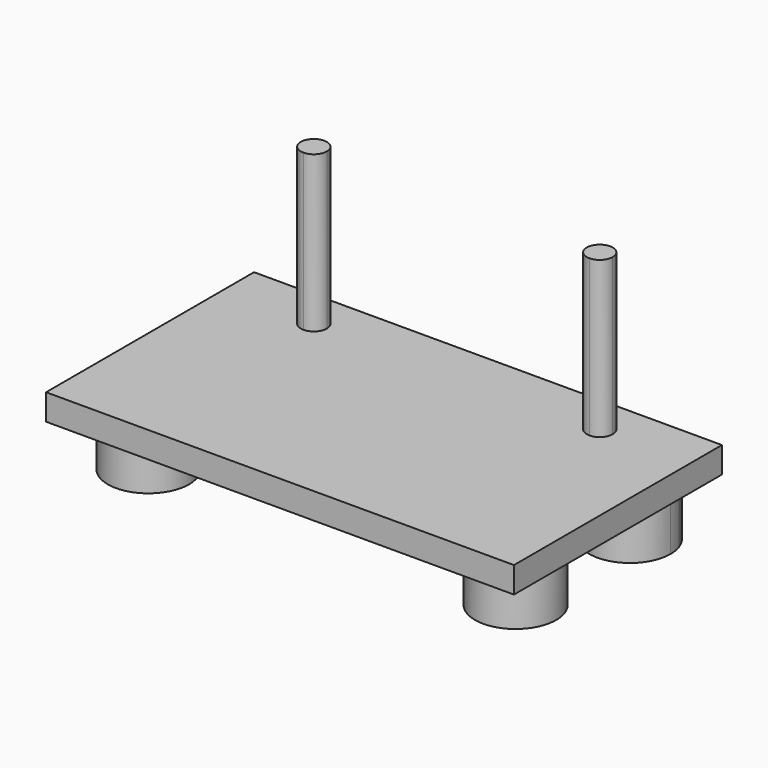
from build123d import *

# Parameters (mm, degrees)
F0_R     = 39.6875
F1_DEPTH = 25.4
F2_DEPTH = 76.2
F3_DEPTH = 152.4


with BuildPart() as f1:
    # F0 (on Top) → F1 (new body)
    with BuildSketch(Plane.XY):
        with BuildLine():
            Line((64.5657867546, -73.7079969396), (0, -73.7079969396))
            Line((0, -73.7079969396), (0, -213.4079969396))
            Line((0, -213.4079969396), (0, -276.9079969396))
            Line((0, -276.9079969396), (228.6, -276.9079969396))
            Line((228.6, -276.9079969396), (228.6, -61.0079969396))
            Line((228.6, -61.0079969396), (216.9881337214, -61.0079969396))
            ThreePointArc((216.9881337214, -61.0079969396), (218.5498084551, -67.2728393878), (219.075, -73.7079969396))
            ThreePointArc((219.075, -73.7079969396), (213.9674206511, -93.1843093218), (199.9593215616, -107.6476170595))
            ThreePointArc((199.9593215616, -107.6476170595), (121.1719117521, -134.9211212537), (64.5657867546, -73.7079969396))
        make_face()
        with BuildLine():
            ThreePointArc((219.075, -213.4079969396), (179.3875, -253.0954969396), (139.7, -213.4079969396))
            ThreePointArc((139.7, -213.4079969396), (179.3875, -173.7204969396), (219.075, -213.4079969396))
        make_face(mode=Mode.SUBTRACT)
        with BuildLine():
            Line((0, -213.4079969396), (0, -73.7079969396))
            Line((0, -73.7079969396), (-64.5657867546, -73.7079969396))
            ThreePointArc((-64.5657867546, -73.7079969396), (-121.1719117521, -134.9211212537), (-199.9593215616, -107.6476170595))
            ThreePointArc((-199.9593215616, -107.6476170595), (-216.6678189317, -87.3195904026), (-216.9881337214, -61.0079969396))
            Line((-216.9881337214, -61.0079969396), (-228.6, -61.0079969396))
            Line((-228.6, -61.0079969396), (-228.6, -276.9079969396))
            Line((-228.6, -276.9079969396), (0, -276.9079969396))
            Line((0, -276.9079969396), (0, -213.4079969396))
        make_face()
        with Locations((-179.3875, -213.4079969396)):
            Circle(F0_R, mode=Mode.SUBTRACT)
        with BuildLine():
            ThreePointArc((219.075, -213.4079969396), (179.3875, -173.7204969396), (139.7, -213.4079969396))
            ThreePointArc((139.7, -213.4079969396), (179.3875, -253.0954969396), (219.075, -213.4079969396))
        make_face()
        with Locations((-179.3875, -213.4079969396)):
            Circle(F0_R)
        with BuildLine():
            ThreePointArc((-199.9593215616, -107.6476170595), (-121.1719117521, -134.9211212537), (-64.5657867546, -73.7079969396))
            Line((-64.5657867546, -73.7079969396), (-125.5009683429, -73.7079969396))
            ThreePointArc((-125.5009683429, -73.7079969396), (-132.1564556102, -78.5007793952), (-140.2101865576, -80.0511639471))
            ThreePointArc((-140.2101865576, -80.0511639471), (-162.7462218601, -109.7380610267), (-199.9593215616, -107.6476170595))
        make_face()
        with BuildLine():
            Line((125.5009683429, -73.7079969396), (64.5657867546, -73.7079969396))
            ThreePointArc((64.5657867546, -73.7079969396), (121.1719117521, -134.9211212537), (199.9593215616, -107.6476170595))
            ThreePointArc((199.9593215616, -107.6476170595), (162.7462218601, -109.7380610267), (140.2101865576, -80.0511639471))
            ThreePointArc((140.2101865576, -80.0511639471), (132.1564556102, -78.5007793952), (125.5009683429, -73.7079969396))
        make_face()
        with BuildLine():
            Line((-158.75, -61.0079969396), (-215.9, -61.0079969396))
            ThreePointArc((-215.9, -61.0079969396), (-211.8047859126, -85.6522629766), (-199.9593215616, -107.6476170595))
            ThreePointArc((-199.9593215616, -107.6476170595), (-162.7462218601, -109.7380610267), (-140.2101865576, -80.0511639471))
            ThreePointArc((-140.2101865576, -80.0511639471), (-147.7093206356, -78.2924779256), (-153.8990316571, -73.7079969396))
            ThreePointArc((-153.8990316571, -73.7079969396), (-157.4959834382, -67.8054577497), (-158.75, -61.0079969396))
        make_face()
        with BuildLine():
            ThreePointArc((199.9593215616, -107.6476170595), (211.8047859126, -85.6522629766), (215.9, -61.0079969396))
            Line((215.9, -61.0079969396), (158.75, -61.0079969396))
            ThreePointArc((158.75, -61.0079969396), (157.4959834382, -67.8054577497), (153.8990316571, -73.7079969396))
            ThreePointArc((153.8990316571, -73.7079969396), (147.7093206356, -78.2924779256), (140.2101865576, -80.0511639471))
            ThreePointArc((140.2101865576, -80.0511639471), (162.7462218601, -109.7380610267), (199.9593215616, -107.6476170595))
        make_face()
        with BuildLine():
            ThreePointArc((-64.2559890942, -50.3009329885), (-67.668281882, -36.1509740894), (-73.7088642316, -22.9079969396))
            Line((-73.7088642316, -22.9079969396), (-205.6911357684, -22.9079969396))
            ThreePointArc((-205.6911357684, -22.9079969396), (-212.902167014, -39.8447565342), (-215.8412589899, -58.0165625961))
            ThreePointArc((-215.8412589899, -58.0165625961), (-186.7550886769, -34.7103522243), (-151.1709455179, -45.7987921962))
            ThreePointArc((-151.1709455179, -45.7987921962), (-144.730628113, -42.6342308371), (-137.5765162555, -42.0767181453))
            Line((-137.5765162555, -42.0767181453), (-64.2559890942, -50.3009329885))
        make_face()
        with BuildLine():
            Line((205.6911357684, -22.9079969396), (73.7088642316, -22.9079969396))
            ThreePointArc((73.7088642316, -22.9079969396), (67.668281882, -36.1509740894), (64.2559890942, -50.3009329885))
            Line((64.2559890942, -50.3009329885), (137.5765161823, -42.0767181535))
            ThreePointArc((137.5765161823, -42.0767181535), (144.7306280775, -42.6342308273), (151.1709455179, -45.7987921962))
            ThreePointArc((151.1709455179, -45.7987921962), (186.7550886769, -34.7103522243), (215.8412589899, -58.0165625961))
            ThreePointArc((215.8412589899, -58.0165625961), (212.902167014, -39.8447565342), (205.6911357684, -22.9079969396))
        make_face()
        with BuildLine():
            Line((0, -22.9079969396), (-73.7088642316, -22.9079969396))
            ThreePointArc((-73.7088642316, -22.9079969396), (-67.668281882, -36.1509740894), (-64.2559890942, -50.3009329885))
            Line((-64.2559890942, -50.3009329885), (0, -57.5083969789))
            Line((0, -57.5083969789), (0, -22.9079969396))
        make_face()
        with BuildLine():
            Line((73.7088642316, -22.9079969396), (0, -22.9079969396))
            Line((0, -22.9079969396), (0, -57.5083969789))
            Line((0, -57.5083969789), (64.2559890942, -50.3009329885))
            ThreePointArc((64.2559890942, -50.3009329885), (67.668281882, -36.1509740894), (73.7088642316, -22.9079969396))
        make_face()
        with BuildLine():
            ThreePointArc((-63.5, -61.0079969396), (-63.6892322397, -55.6411371043), (-64.2559890942, -50.3009329885))
            Line((-64.2559890942, -50.3009329885), (-137.5765162555, -42.0767181453))
            ThreePointArc((-137.5765162555, -42.0767181453), (-125.4986820095, -48.3105536011), (-120.65, -61.0079969396))
            ThreePointArc((-120.65, -61.0079969396), (-121.9040165618, -67.8054577497), (-125.5009683429, -73.7079969396))
            Line((-125.5009683429, -73.7079969396), (-64.5657867546, -73.7079969396))
            ThreePointArc((-64.5657867546, -73.7079969396), (-63.7669141635, -67.3803179729), (-63.5, -61.0079969396))
        make_face()
        with BuildLine():
            Line((137.5765161823, -42.0767181535), (64.2559890942, -50.3009329885))
            ThreePointArc((64.2559890942, -50.3009329885), (63.5066731411, -62.0164324464), (64.5657867546, -73.7079969396))
            Line((64.5657867546, -73.7079969396), (125.5009683429, -73.7079969396))
            ThreePointArc((125.5009683429, -73.7079969396), (121.9027929925, -54.2137403406), (137.5765161823, -42.0767181535))
        make_face()
        with BuildLine():
            ThreePointArc((-151.1709455179, -45.7987921962), (-186.7550886769, -34.7103522243), (-215.8412589899, -58.0165625961))
            ThreePointArc((-215.8412589899, -58.0165625961), (-215.8853133321, -59.5119914301), (-215.9, -61.0079969396))
            Line((-215.9, -61.0079969396), (-158.75, -61.0079969396))
            ThreePointArc((-158.75, -61.0079969396), (-156.7502787677, -52.5114980169), (-151.1709455179, -45.7987921962))
        make_face()
        with BuildLine():
            ThreePointArc((215.9, -61.0079969396), (215.8853133321, -59.5119914301), (215.8412589899, -58.0165625961))
            ThreePointArc((215.8412589899, -58.0165625961), (186.7550886769, -34.7103522243), (151.1709455179, -45.7987921962))
            ThreePointArc((151.1709455179, -45.7987921962), (156.7502787677, -52.5114980169), (158.75, -61.0079969396))
            Line((158.75, -61.0079969396), (215.9, -61.0079969396))
        make_face()
        with BuildLine():
            Line((0, -57.5083969789), (-64.2559890942, -50.3009329885))
            ThreePointArc((-64.2559890942, -50.3009329885), (-63.6892322397, -55.6411371043), (-63.5, -61.0079969396))
            ThreePointArc((-63.5, -61.0079969396), (-63.7669141635, -67.3803179729), (-64.5657867546, -73.7079969396))
            Line((-64.5657867546, -73.7079969396), (0, -73.7079969396))
            Line((0, -73.7079969396), (0, -57.5083969789))
        make_face()
        with BuildLine():
            Line((64.2559890942, -50.3009329885), (0, -57.5083969789))
            Line((0, -57.5083969789), (0, -73.7079969396))
            Line((0, -73.7079969396), (64.5657867546, -73.7079969396))
            ThreePointArc((64.5657867546, -73.7079969396), (63.5066731411, -62.0164324464), (64.2559890942, -50.3009329885))
        make_face()
        with BuildLine():
            ThreePointArc((-215.8412589899, -58.0165625961), (-212.902167014, -39.8447565342), (-205.6911357684, -22.9079969396))
            Line((-205.6911357684, -22.9079969396), (-228.6, -22.9079969396))
            Line((-228.6, -22.9079969396), (-228.6, -61.0079969396))
            Line((-228.6, -61.0079969396), (-216.9881337214, -61.0079969396))
            ThreePointArc((-216.9881337214, -61.0079969396), (-216.4448938617, -59.5007024599), (-215.8412589899, -58.0165625961))
        make_face()
        with BuildLine():
            Line((228.6, -22.9079969396), (205.6911357684, -22.9079969396))
            ThreePointArc((205.6911357684, -22.9079969396), (212.902167014, -39.8447565342), (215.8412589899, -58.0165625961))
            ThreePointArc((215.8412589899, -58.0165625961), (216.4448938617, -59.5007024599), (216.9881337214, -61.0079969396))
            Line((216.9881337214, -61.0079969396), (228.6, -61.0079969396))
            Line((228.6, -61.0079969396), (228.6, -22.9079969396))
        make_face()
        with BuildLine():
            ThreePointArc((-127, -61.0079969396), (-133.8839513111, -49.7180200729), (-147.0730043541, -50.6673583329))
            ThreePointArc((-147.0730043541, -50.6673583329), (-144.0496515891, -55.6432764617), (-141.7868662786, -61.0079969396))
            ThreePointArc((-141.7868662786, -61.0079969396), (-140.2251915449, -67.2728393878), (-139.7, -73.7079969396))
            ThreePointArc((-139.7, -73.7079969396), (-130.7197438789, -69.9882530606), (-127, -61.0079969396))
        make_face()
        with BuildLine():
            ThreePointArc((141.7868662786, -61.0079969396), (144.0496515891, -55.6432764617), (147.0730043541, -50.6673583329))
            ThreePointArc((147.0730043541, -50.6673583329), (127.6042133306, -57.1373452053), (139.7, -73.7079969396))
            ThreePointArc((139.7, -73.7079969396), (140.2251915449, -67.2728393878), (141.7868662786, -61.0079969396))
        make_face()
        with BuildLine():
            ThreePointArc((-120.65, -61.0079969396), (-125.4986820095, -48.3105536011), (-137.5765162555, -42.0767181453))
            ThreePointArc((-137.5765162555, -42.0767181453), (-144.730628113, -42.6342308371), (-151.1709455179, -45.7987921962))
            ThreePointArc((-151.1709455179, -45.7987921962), (-149.0242369761, -48.1508078376), (-147.0730043541, -50.6673583329))
            ThreePointArc((-147.0730043541, -50.6673583329), (-133.8839513111, -49.7180200729), (-127, -61.0079969396))
            ThreePointArc((-127, -61.0079969396), (-130.7197438789, -69.9882530606), (-139.7, -73.7079969396))
            Line((-139.7, -73.7079969396), (-125.5009683429, -73.7079969396))
            ThreePointArc((-125.5009683429, -73.7079969396), (-121.9040165618, -67.8054577497), (-120.65, -61.0079969396))
        make_face()
        with BuildLine():
            ThreePointArc((151.1709455179, -45.7987921962), (144.7306280775, -42.6342308273), (137.5765161823, -42.0767181535))
            ThreePointArc((137.5765161823, -42.0767181535), (121.9027929925, -54.2137403406), (125.5009683429, -73.7079969396))
            Line((125.5009683429, -73.7079969396), (139.7, -73.7079969396))
            ThreePointArc((139.7, -73.7079969396), (127.6042133306, -57.1373452053), (147.0730043541, -50.6673583329))
            ThreePointArc((147.0730043541, -50.6673583329), (149.0242369761, -48.1508078376), (151.1709455179, -45.7987921962))
        make_face()
        with BuildLine():
            ThreePointArc((-199.9593215616, -107.6476170595), (-211.8047859126, -85.6522629766), (-215.9, -61.0079969396))
            Line((-215.9, -61.0079969396), (-216.9881337214, -61.0079969396))
            ThreePointArc((-216.9881337214, -61.0079969396), (-216.6678189317, -87.3195904026), (-199.9593215616, -107.6476170595))
        make_face()
        with BuildLine():
            Line((216.9881337214, -61.0079969396), (215.9, -61.0079969396))
            ThreePointArc((215.9, -61.0079969396), (211.8047859126, -85.6522629766), (199.9593215616, -107.6476170595))
            ThreePointArc((199.9593215616, -107.6476170595), (213.9674206511, -93.1843093218), (219.075, -73.7079969396))
            ThreePointArc((219.075, -73.7079969396), (218.5498084551, -67.2728393878), (216.9881337214, -61.0079969396))
        make_face()
        with BuildLine():
            ThreePointArc((-152.4, -61.0079969396), (-148.6802561211, -69.9882530606), (-139.7, -73.7079969396))
            ThreePointArc((-139.7, -73.7079969396), (-140.2251915449, -67.2728393878), (-141.7868662786, -61.0079969396))
            Line((-141.7868662786, -61.0079969396), (-152.4, -61.0079969396))
        make_face()
        with BuildLine():
            ThreePointArc((141.7868662786, -61.0079969396), (140.2251915449, -67.2728393878), (139.7, -73.7079969396))
            ThreePointArc((139.7, -73.7079969396), (148.6802561211, -69.9882530606), (152.4, -61.0079969396))
            Line((152.4, -61.0079969396), (141.7868662786, -61.0079969396))
        make_face()
        with BuildLine():
            Line((-152.4, -61.0079969396), (-158.75, -61.0079969396))
            ThreePointArc((-158.75, -61.0079969396), (-157.4959834382, -67.8054577497), (-153.8990316571, -73.7079969396))
            Line((-153.8990316571, -73.7079969396), (-139.7, -73.7079969396))
            ThreePointArc((-139.7, -73.7079969396), (-148.6802561211, -69.9882530606), (-152.4, -61.0079969396))
        make_face()
        with BuildLine():
            ThreePointArc((153.8990316571, -73.7079969396), (157.4959834382, -67.8054577497), (158.75, -61.0079969396))
            Line((158.75, -61.0079969396), (152.4, -61.0079969396))
            ThreePointArc((152.4, -61.0079969396), (148.6802561211, -69.9882530606), (139.7, -73.7079969396))
            Line((139.7, -73.7079969396), (153.8990316571, -73.7079969396))
        make_face()
        with BuildLine():
            ThreePointArc((-147.0730043541, -50.6673583329), (-149.0242369761, -48.1508078376), (-151.1709455179, -45.7987921962))
            ThreePointArc((-151.1709455179, -45.7987921962), (-156.7502787677, -52.5114980169), (-158.75, -61.0079969396))
            Line((-158.75, -61.0079969396), (-152.4, -61.0079969396))
            ThreePointArc((-152.4, -61.0079969396), (-150.9899768666, -55.1919482507), (-147.0730043541, -50.6673583329))
        make_face()
        with BuildLine():
            ThreePointArc((158.75, -61.0079969396), (156.7502787677, -52.5114980169), (151.1709455179, -45.7987921962))
            ThreePointArc((151.1709455179, -45.7987921962), (149.0242369761, -48.1508078376), (147.0730043541, -50.6673583329))
            ThreePointArc((147.0730043541, -50.6673583329), (150.9899768666, -55.1919482507), (152.4, -61.0079969396))
            Line((152.4, -61.0079969396), (158.75, -61.0079969396))
        make_face()
        with BuildLine():
            ThreePointArc((-141.7868662786, -61.0079969396), (-144.0496515891, -55.6432764617), (-147.0730043541, -50.6673583329))
            ThreePointArc((-147.0730043541, -50.6673583329), (-150.9899768666, -55.1919482507), (-152.4, -61.0079969396))
            Line((-152.4, -61.0079969396), (-141.7868662786, -61.0079969396))
        make_face()
        with BuildLine():
            ThreePointArc((152.4, -61.0079969396), (150.9899768666, -55.1919482507), (147.0730043541, -50.6673583329))
            ThreePointArc((147.0730043541, -50.6673583329), (144.0496515891, -55.6432764617), (141.7868662786, -61.0079969396))
            Line((141.7868662786, -61.0079969396), (152.4, -61.0079969396))
        make_face()
        with BuildLine():
            ThreePointArc((-140.2101865576, -80.0511639471), (-132.1564556102, -78.5007793952), (-125.5009683429, -73.7079969396))
            Line((-125.5009683429, -73.7079969396), (-139.7, -73.7079969396))
            ThreePointArc((-139.7, -73.7079969396), (-139.8277522537, -76.8898225951), (-140.2101865576, -80.0511639471))
        make_face()
        with BuildLine():
            Line((139.7, -73.7079969396), (125.5009683429, -73.7079969396))
            ThreePointArc((125.5009683429, -73.7079969396), (132.1564556102, -78.5007793952), (140.2101865576, -80.0511639471))
            ThreePointArc((140.2101865576, -80.0511639471), (139.8277522537, -76.8898225951), (139.7, -73.7079969396))
        make_face()
        with BuildLine():
            ThreePointArc((-153.8990316571, -73.7079969396), (-147.7093206356, -78.2924779256), (-140.2101865576, -80.0511639471))
            ThreePointArc((-140.2101865576, -80.0511639471), (-139.8277522537, -76.8898225951), (-139.7, -73.7079969396))
            Line((-139.7, -73.7079969396), (-153.8990316571, -73.7079969396))
        make_face()
        with BuildLine():
            ThreePointArc((139.7, -73.7079969396), (139.8277522537, -76.8898225951), (140.2101865576, -80.0511639471))
            ThreePointArc((140.2101865576, -80.0511639471), (147.7093206356, -78.2924779256), (153.8990316571, -73.7079969396))
            Line((153.8990316571, -73.7079969396), (139.7, -73.7079969396))
        make_face()
        with BuildLine():
            ThreePointArc((-215.9, -61.0079969396), (-215.8853133321, -59.5119914301), (-215.8412589899, -58.0165625961))
            ThreePointArc((-215.8412589899, -58.0165625961), (-216.4448938617, -59.5007024599), (-216.9881337214, -61.0079969396))
            Line((-216.9881337214, -61.0079969396), (-215.9, -61.0079969396))
        make_face()
    extrude(amount=-F1_DEPTH)

    # F0 (on Top) → F2 (join)
    with BuildSketch(Plane.XY):
        with BuildLine():
            ThreePointArc((-151.1709455179, -45.7987921962), (-186.7550886769, -34.7103522243), (-215.8412589899, -58.0165625961))
            ThreePointArc((-215.8412589899, -58.0165625961), (-215.8853133321, -59.5119914301), (-215.9, -61.0079969396))
            Line((-215.9, -61.0079969396), (-158.75, -61.0079969396))
            ThreePointArc((-158.75, -61.0079969396), (-156.7502787677, -52.5114980169), (-151.1709455179, -45.7987921962))
        make_face()
        with BuildLine():
            ThreePointArc((-215.9, -61.0079969396), (-215.8853133321, -59.5119914301), (-215.8412589899, -58.0165625961))
            ThreePointArc((-215.8412589899, -58.0165625961), (-216.4448938617, -59.5007024599), (-216.9881337214, -61.0079969396))
            Line((-216.9881337214, -61.0079969396), (-215.9, -61.0079969396))
        make_face()
        with BuildLine():
            ThreePointArc((219.075, -213.4079969396), (179.3875, -173.7204969396), (139.7, -213.4079969396))
            ThreePointArc((139.7, -213.4079969396), (179.3875, -253.0954969396), (219.075, -213.4079969396))
        make_face()
        with Locations((-179.3875, -213.4079969396)):
            Circle(F0_R)
        with BuildLine():
            ThreePointArc((-147.0730043541, -50.6673583329), (-149.0242369761, -48.1508078376), (-151.1709455179, -45.7987921962))
            ThreePointArc((-151.1709455179, -45.7987921962), (-156.7502787677, -52.5114980169), (-158.75, -61.0079969396))
            Line((-158.75, -61.0079969396), (-152.4, -61.0079969396))
            ThreePointArc((-152.4, -61.0079969396), (-150.9899768666, -55.1919482507), (-147.0730043541, -50.6673583329))
        make_face()
        with BuildLine():
            Line((-158.75, -61.0079969396), (-215.9, -61.0079969396))
            ThreePointArc((-215.9, -61.0079969396), (-211.8047859126, -85.6522629766), (-199.9593215616, -107.6476170595))
            ThreePointArc((-199.9593215616, -107.6476170595), (-162.7462218601, -109.7380610267), (-140.2101865576, -80.0511639471))
            ThreePointArc((-140.2101865576, -80.0511639471), (-147.7093206356, -78.2924779256), (-153.8990316571, -73.7079969396))
            ThreePointArc((-153.8990316571, -73.7079969396), (-157.4959834382, -67.8054577497), (-158.75, -61.0079969396))
        make_face()
        with BuildLine():
            ThreePointArc((-199.9593215616, -107.6476170595), (-211.8047859126, -85.6522629766), (-215.9, -61.0079969396))
            Line((-215.9, -61.0079969396), (-216.9881337214, -61.0079969396))
            ThreePointArc((-216.9881337214, -61.0079969396), (-216.6678189317, -87.3195904026), (-199.9593215616, -107.6476170595))
        make_face()
        with BuildLine():
            ThreePointArc((216.9881337214, -61.0079969396), (216.4448938617, -59.5007024599), (215.8412589899, -58.0165625961))
            ThreePointArc((215.8412589899, -58.0165625961), (215.8853133321, -59.5119914301), (215.9, -61.0079969396))
            Line((215.9, -61.0079969396), (216.9881337214, -61.0079969396))
        make_face()
        with BuildLine():
            ThreePointArc((215.9, -61.0079969396), (215.8853133321, -59.5119914301), (215.8412589899, -58.0165625961))
            ThreePointArc((215.8412589899, -58.0165625961), (186.7550886769, -34.7103522243), (151.1709455179, -45.7987921962))
            ThreePointArc((151.1709455179, -45.7987921962), (156.7502787677, -52.5114980169), (158.75, -61.0079969396))
            Line((158.75, -61.0079969396), (215.9, -61.0079969396))
        make_face()
        with BuildLine():
            Line((-152.4, -61.0079969396), (-158.75, -61.0079969396))
            ThreePointArc((-158.75, -61.0079969396), (-157.4959834382, -67.8054577497), (-153.8990316571, -73.7079969396))
            Line((-153.8990316571, -73.7079969396), (-139.7, -73.7079969396))
            ThreePointArc((-139.7, -73.7079969396), (-148.6802561211, -69.9882530606), (-152.4, -61.0079969396))
        make_face()
        with BuildLine():
            ThreePointArc((-141.7868662786, -61.0079969396), (-144.0496515891, -55.6432764617), (-147.0730043541, -50.6673583329))
            ThreePointArc((-147.0730043541, -50.6673583329), (-150.9899768666, -55.1919482507), (-152.4, -61.0079969396))
            Line((-152.4, -61.0079969396), (-141.7868662786, -61.0079969396))
        make_face()
        with BuildLine():
            Line((216.9881337214, -61.0079969396), (215.9, -61.0079969396))
            ThreePointArc((215.9, -61.0079969396), (211.8047859126, -85.6522629766), (199.9593215616, -107.6476170595))
            ThreePointArc((199.9593215616, -107.6476170595), (213.9674206511, -93.1843093218), (219.075, -73.7079969396))
            ThreePointArc((219.075, -73.7079969396), (218.5498084551, -67.2728393878), (216.9881337214, -61.0079969396))
        make_face()
        with BuildLine():
            ThreePointArc((199.9593215616, -107.6476170595), (211.8047859126, -85.6522629766), (215.9, -61.0079969396))
            Line((215.9, -61.0079969396), (158.75, -61.0079969396))
            ThreePointArc((158.75, -61.0079969396), (157.4959834382, -67.8054577497), (153.8990316571, -73.7079969396))
            ThreePointArc((153.8990316571, -73.7079969396), (147.7093206356, -78.2924779256), (140.2101865576, -80.0511639471))
            ThreePointArc((140.2101865576, -80.0511639471), (162.7462218601, -109.7380610267), (199.9593215616, -107.6476170595))
        make_face()
        with BuildLine():
            ThreePointArc((158.75, -61.0079969396), (156.7502787677, -52.5114980169), (151.1709455179, -45.7987921962))
            ThreePointArc((151.1709455179, -45.7987921962), (149.0242369761, -48.1508078376), (147.0730043541, -50.6673583329))
            ThreePointArc((147.0730043541, -50.6673583329), (150.9899768666, -55.1919482507), (152.4, -61.0079969396))
            Line((152.4, -61.0079969396), (158.75, -61.0079969396))
        make_face()
        with BuildLine():
            ThreePointArc((-153.8990316571, -73.7079969396), (-147.7093206356, -78.2924779256), (-140.2101865576, -80.0511639471))
            ThreePointArc((-140.2101865576, -80.0511639471), (-139.8277522537, -76.8898225951), (-139.7, -73.7079969396))
            Line((-139.7, -73.7079969396), (-153.8990316571, -73.7079969396))
        make_face()
        with BuildLine():
            ThreePointArc((-152.4, -61.0079969396), (-148.6802561211, -69.9882530606), (-139.7, -73.7079969396))
            ThreePointArc((-139.7, -73.7079969396), (-140.2251915449, -67.2728393878), (-141.7868662786, -61.0079969396))
            Line((-141.7868662786, -61.0079969396), (-152.4, -61.0079969396))
        make_face()
        with BuildLine():
            ThreePointArc((153.8990316571, -73.7079969396), (157.4959834382, -67.8054577497), (158.75, -61.0079969396))
            Line((158.75, -61.0079969396), (152.4, -61.0079969396))
            ThreePointArc((152.4, -61.0079969396), (148.6802561211, -69.9882530606), (139.7, -73.7079969396))
            Line((139.7, -73.7079969396), (153.8990316571, -73.7079969396))
        make_face()
        with BuildLine():
            ThreePointArc((152.4, -61.0079969396), (150.9899768666, -55.1919482507), (147.0730043541, -50.6673583329))
            ThreePointArc((147.0730043541, -50.6673583329), (144.0496515891, -55.6432764617), (141.7868662786, -61.0079969396))
            Line((141.7868662786, -61.0079969396), (152.4, -61.0079969396))
        make_face()
        with BuildLine():
            ThreePointArc((139.7, -73.7079969396), (139.8277522537, -76.8898225951), (140.2101865576, -80.0511639471))
            ThreePointArc((140.2101865576, -80.0511639471), (147.7093206356, -78.2924779256), (153.8990316571, -73.7079969396))
            Line((153.8990316571, -73.7079969396), (139.7, -73.7079969396))
        make_face()
        with BuildLine():
            ThreePointArc((141.7868662786, -61.0079969396), (140.2251915449, -67.2728393878), (139.7, -73.7079969396))
            ThreePointArc((139.7, -73.7079969396), (148.6802561211, -69.9882530606), (152.4, -61.0079969396))
            Line((152.4, -61.0079969396), (141.7868662786, -61.0079969396))
        make_face()
    extrude(amount=-F2_DEPTH)

    # F0 (on Top) → F3 (join)
    with BuildSketch(Plane.XY):
        with BuildLine():
            ThreePointArc((-141.7868662786, -61.0079969396), (-144.0496515891, -55.6432764617), (-147.0730043541, -50.6673583329))
            ThreePointArc((-147.0730043541, -50.6673583329), (-150.9899768666, -55.1919482507), (-152.4, -61.0079969396))
            Line((-152.4, -61.0079969396), (-141.7868662786, -61.0079969396))
        make_face()
        with BuildLine():
            ThreePointArc((-152.4, -61.0079969396), (-148.6802561211, -69.9882530606), (-139.7, -73.7079969396))
            ThreePointArc((-139.7, -73.7079969396), (-140.2251915449, -67.2728393878), (-141.7868662786, -61.0079969396))
            Line((-141.7868662786, -61.0079969396), (-152.4, -61.0079969396))
        make_face()
        with BuildLine():
            ThreePointArc((-127, -61.0079969396), (-133.8839513111, -49.7180200729), (-147.0730043541, -50.6673583329))
            ThreePointArc((-147.0730043541, -50.6673583329), (-144.0496515891, -55.6432764617), (-141.7868662786, -61.0079969396))
            ThreePointArc((-141.7868662786, -61.0079969396), (-140.2251915449, -67.2728393878), (-139.7, -73.7079969396))
            ThreePointArc((-139.7, -73.7079969396), (-130.7197438789, -69.9882530606), (-127, -61.0079969396))
        make_face()
        with BuildLine():
            ThreePointArc((152.4, -61.0079969396), (150.9899768666, -55.1919482507), (147.0730043541, -50.6673583329))
            ThreePointArc((147.0730043541, -50.6673583329), (144.0496515891, -55.6432764617), (141.7868662786, -61.0079969396))
            Line((141.7868662786, -61.0079969396), (152.4, -61.0079969396))
        make_face()
        with BuildLine():
            ThreePointArc((141.7868662786, -61.0079969396), (144.0496515891, -55.6432764617), (147.0730043541, -50.6673583329))
            ThreePointArc((147.0730043541, -50.6673583329), (127.6042133306, -57.1373452053), (139.7, -73.7079969396))
            ThreePointArc((139.7, -73.7079969396), (140.2251915449, -67.2728393878), (141.7868662786, -61.0079969396))
        make_face()
        with BuildLine():
            ThreePointArc((141.7868662786, -61.0079969396), (140.2251915449, -67.2728393878), (139.7, -73.7079969396))
            ThreePointArc((139.7, -73.7079969396), (148.6802561211, -69.9882530606), (152.4, -61.0079969396))
            Line((152.4, -61.0079969396), (141.7868662786, -61.0079969396))
        make_face()
    extrude(amount=F3_DEPTH)


solid = f1.part
